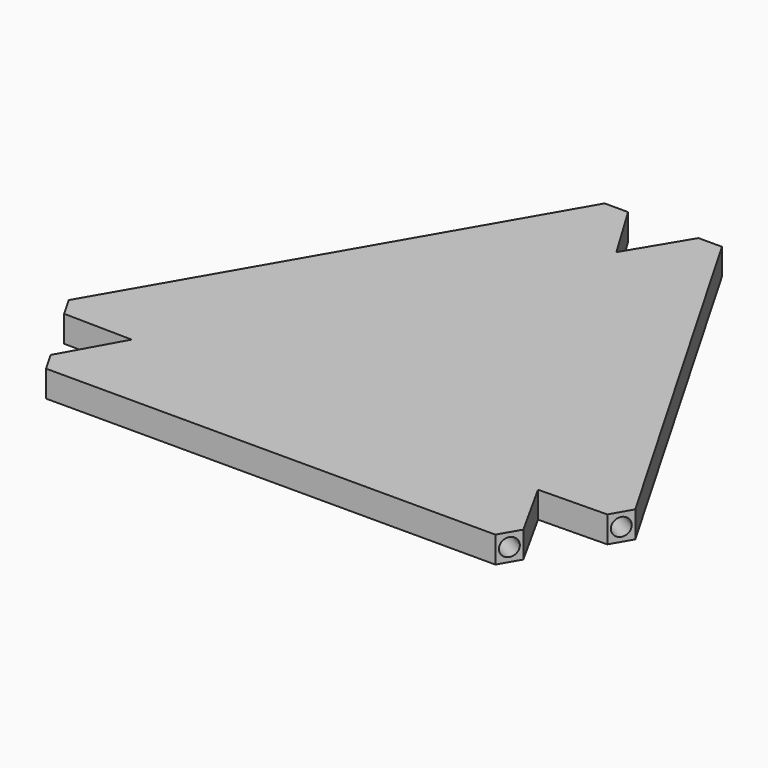
from build123d import *

# Parameters (mm, degrees)
F1_DEPTH       = 2.25
F1_DEPTH_BACK  = 2.25
F3_DEPTH       = 20
F10_DEPTH      = 2.251
F10_DEPTH_BACK = 25


# Not quite as in the source:
# - a feature names something its author has since deleted; it is built from what else it names


with BuildPart() as f1:
    # F0 (on Top) → F1 (new body, two sides)
    with BuildSketch(Plane.XY) as f1_sk:
        Polygon((10, 50), (0, 50), (21.6506350946, 12.5), (29.1506350946, 16.8301270189), align=None)
        Polygon((-21.6506350946, 12.5), (0, 50), (-10, 50), (-29.1506350946, 16.8301270189), align=None)
        Polygon((21.6506350946, 12.5), (0, 50), (0, 0), align=None)
        Polygon((0, 0), (0, 50), (-21.6506350946, 12.5), align=None)
        Polygon((29.1506350946, 16.8301270189), (21.6506350946, 12.5), (43.3012701892, -25), (48.3012701892, -16.3397459622), align=None)
        Polygon((43.3012701892, -25), (21.6506350946, 12.5), (0, 0), align=None)
        Polygon((43.3012701892, -25), (0, 0), (-43.3012701892, -25), align=None)
        Polygon((-43.3012701892, -25), (0, 0), (-21.6506350946, 12.5), align=None)
        Polygon((-43.3012701892, -25), (-21.6506350946, 12.5), (-29.1506350946, 16.8301270189), (-48.3012701892, -16.3397459622), align=None)
        Polygon((38.3012701892, -33.6602540378), (43.3012701892, -25), (-43.3012701892, -25), (-38.3012701892, -33.6602540378), align=None)
    extrude(amount=F1_DEPTH)
    extrude(f1_sk.sketch, amount=-F1_DEPTH_BACK)


with BuildPart() as f3:
    # F2 (on face) → F3 (new body)
    with BuildSketch(Plane(origin=(0, 50, 0), x_dir=(-1, 0, 0), z_dir=(0, 1, 0))):
        with BuildLine():
            Line((-8, 0), (-6.5, 0))
            ThreePointArc((-6.5, 0), (-6.9393398282, 1.0606601718), (-8, 1.5))
            Line((-8, 1.5), (-8, 0))
        make_face()
        with BuildLine():
            ThreePointArc((-9.5, 0), (-8, -1.5), (-6.5, 0))
            Line((-6.5, 0), (-8, 0))
            Line((-8, 0), (-9.5, 0))
        make_face()
        with BuildLine():
            Line((-8, 0), (-8, 1.5))
            ThreePointArc((-8, 1.5), (-9.0606601718, 1.0606601718), (-9.5, 0))
            Line((-9.5, 0), (-8, 0))
        make_face()
    extrude(amount=-F3_DEPTH)


with BuildPart() as f3b:
    # F2 (on face) → F3, piece 2 (new body)
    with BuildSketch(Plane(origin=(0, 50, 0), x_dir=(-1, 0, 0), z_dir=(0, 1, 0))):
        with BuildLine():
            ThreePointArc((8, 1.5), (6.9393398282, 1.0606601718), (6.5, 0))
            Line((6.5, 0), (8, 0))
            Line((8, 0), (8, 1.5))
        make_face()
        with BuildLine():
            Line((8, 0), (6.5, 0))
            ThreePointArc((6.5, 0), (8, -1.5), (9.5, 0))
            Line((9.5, 0), (8, 0))
        make_face()
        with BuildLine():
            ThreePointArc((9.5, 0), (9.0606601718, 1.0606601718), (8, 1.5))
            Line((8, 1.5), (8, 0))
            Line((8, 0), (9.5, 0))
        make_face()
    extrude(amount=-F3_DEPTH)


with BuildPart() as f6_1:
    # F6: instance of F3
    add(f3.part.mirror(Plane(origin=(0, 0, 0), x_dir=(0.8660254038, 0.5, 0), z_dir=(0.5, -0.8660254038, 0))))


with BuildPart() as f6_2:
    # F6: instance of F3b
    add(f3b.part.mirror(Plane(origin=(0, 0, 0), x_dir=(0.8660254038, 0.5, 0), z_dir=(0.5, -0.8660254038, 0))))


with BuildPart() as f7_1:
    # F7: instance of F3
    add(f3.part.mirror(Plane(origin=(0, 0, 0), x_dir=(0.8660254038, -0.5, 0), z_dir=(-0.5, -0.8660254038, 0))))


with BuildPart() as f7_2:
    # F7: instance of F3b
    add(f3b.part.mirror(Plane(origin=(0, 0, 0), x_dir=(0.8660254038, -0.5, 0), z_dir=(-0.5, -0.8660254038, 0))))


with BuildPart() as f1_1:
    add(f1.part)

    # F8: cut F3, F3b, F6_1, F6_2, F7_2, F7_1
    add(f3.part, mode=Mode.SUBTRACT)
    add(f3b.part, mode=Mode.SUBTRACT)
    add(f6_1.part, mode=Mode.SUBTRACT)
    add(f6_2.part, mode=Mode.SUBTRACT)
    add(f7_2.part, mode=Mode.SUBTRACT)
    add(f7_1.part, mode=Mode.SUBTRACT)

    # F9 (on Top) → F10 (cut, two sides)
    with BuildSketch(Plane.XY) as f10_sk:
        Polygon((0, 50), (-6, 50), (0, 40), align=None)
        Polygon((0, 50), (0, 40), (6, 50), align=None)
        Polygon((-40.3012701892, -30.1961524227), (-34.6410161514, -20), (-43.3012701892, -25), align=None)
        Polygon((-43.3012701892, -25), (-34.6410161514, -20), (-46.3012701892, -19.8038475773), align=None)
        Polygon((34.6410161514, -20), (43.3012701892, -25), (46.3012701892, -19.8038475773), align=None)
        Polygon((40.3012701892, -30.1961524227), (43.3012701892, -25), (34.6410161514, -20), align=None)
    extrude(amount=-F10_DEPTH, mode=Mode.SUBTRACT)
    extrude(f10_sk.sketch, amount=F10_DEPTH_BACK, mode=Mode.SUBTRACT)


solid = f1_1.part
